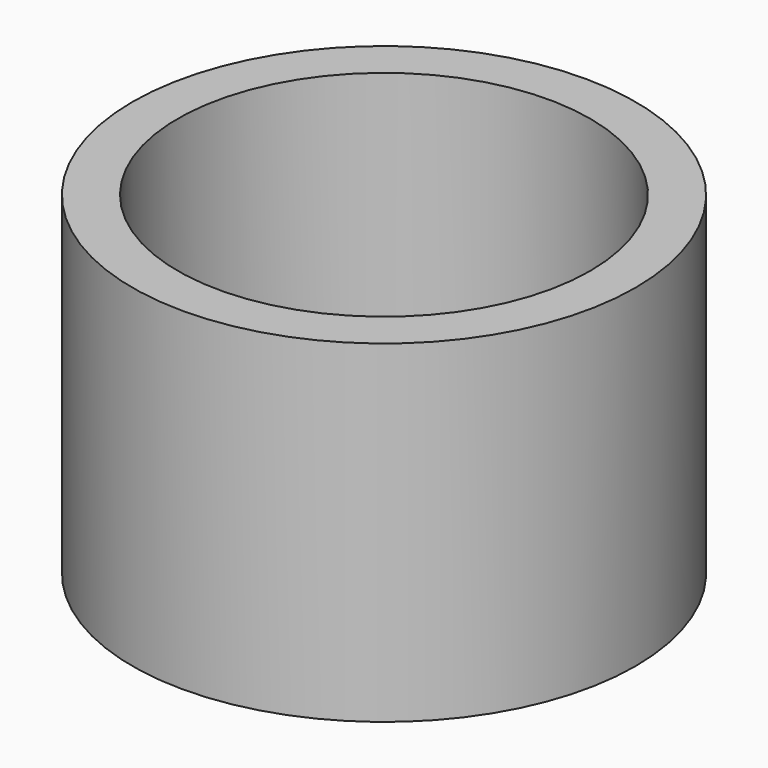
from build123d import *

# Parameters (mm, degrees)
F0_R     = 19.1787076441
F1_DEPTH = 25.4
F6_R     = 15.7197255207
F7_DEPTH = 19.05


# Not quite as in the source:
# - the program builds the solid bodies; features that only make, move or delete a surface that nothing else refers to are left out


with BuildPart() as f1:
    # F0 (on Top) → F1 (new body)
    with BuildSketch(Plane.XY):
        Circle(F0_R)
    extrude(amount=F1_DEPTH)

    # F6 (on face) → F7 (cut)
    with BuildSketch(Plane.XY.offset(25.4)):
        Circle(F6_R)
    extrude(amount=-F7_DEPTH, mode=Mode.SUBTRACT)


solid = f1.part
